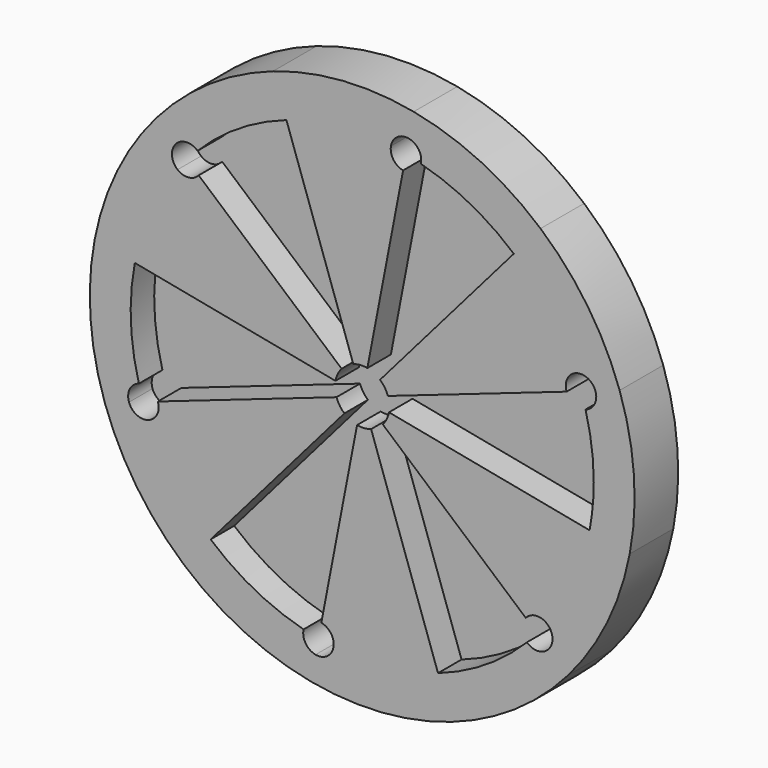
from build123d import *

# Parameters (mm, degrees)
F1_DEPTH = 12.7
F2_R     = 63.5
F3_DEPTH = 5.842


# Not quite as in the source:
# - a feature names something its author has since deleted; it is built from what else it names


with BuildPart() as f1:
    # F0 (on Front) → F1 (new body)
    with BuildSketch(Plane.XZ):
        with BuildLine():
            Line((54.3616852417, 18.8314401648), (60.0018600902, 20.785254045))
            ThreePointArc((60.0018600902, 20.785254045), (52.5777266824, 35.6066378209), (41.57050809, 48.0014880722))
            Line((41.57050809, 48.0014880722), (35.3349318765, 40.8012648613))
            ThreePointArc((35.3349318765, 40.8012648613), (43.6698276291, 31.7213930943), (49.7275527638, 20.9874038681))
            ThreePointArc((49.7275527638, 20.9874038681), (52.5015720726, 20.8916190072), (54.3616852417, 18.8314401648))
        make_face()
        with BuildLine():
            Line((35.3349318765, 40.8012648613), (41.57050809, 48.0014880722))
            ThreePointArc((41.57050809, 48.0014880722), (27.7303280697, 57.1251162375), (12.000372018, 62.3557621349))
            Line((12.000372018, 62.3557621349), (10.8723370483, 56.4943204943))
            ThreePointArc((10.8723370483, 56.4943204943), (12.9421077904, 55.2668436539), (13.7563162153, 53.0023978147))
            ThreePointArc((13.7563162153, 53.0023978147), (13.7342201731, 52.6065963274), (13.6682066443, 52.2157136514))
            ThreePointArc((13.6682066443, 52.2157136514), (25.1574900679, 47.7535477057), (35.3349318765, 40.8012648613))
        make_face()
        with BuildLine():
            Line((10.8723370483, 56.4943204943), (12.000372018, 62.3557621349))
            ThreePointArc((12.000372018, 62.3557621349), (-4.5473895551, 63.3369658907), (-20.785254045, 60.0018600902))
            Line((-20.785254045, 60.0018600902), (-17.6674659382, 51.0015810767))
            ThreePointArc((-17.6674659382, 51.0015810767), (-5.6366184485, 53.6798766529), (6.6881514727, 53.5590258955))
            ThreePointArc((6.6881514727, 53.5590258955), (8.1581132499, 55.9135046571), (10.8723370483, 56.4943204943))
        make_face()
        with BuildLine():
            Line((-17.6674659382, 51.0015810767), (-20.785254045, 60.0018600902))
            ThreePointArc((-20.785254045, 60.0018600902), (-35.6066378209, 52.5777266824), (-48.0014880722, 41.57050809))
            Line((-48.0014880722, 41.57050809), (-43.4893481934, 37.6628803295))
            ThreePointArc((-43.4893481934, 37.6628803295), (-40.9974571589, 38.8855155725), (-38.3860311767, 37.9448710039))
            ThreePointArc((-38.3860311767, 37.9448710039), (-28.7770404, 45.6637993471), (-17.6674659382, 51.0015810767))
        make_face()
        with BuildLine():
            Line((-43.4893481934, 37.6628803295), (-48.0014880722, 41.57050809))
            ThreePointArc((-48.0014880722, 41.57050809), (-57.1251162375, 27.7303280697), (-62.3557621349, 12.000372018))
            Line((-62.3557621349, 12.000372018), (-53.0023978147, 10.2003162153))
            ThreePointArc((-53.0023978147, 10.2003162153), (-49.3064460776, 21.9584835586), (-43.0394012911, 32.5716220275))
            ThreePointArc((-43.0394012911, 32.5716220275), (-44.3434588227, 35.0218856499), (-43.4893481934, 37.6628803295))
        make_face()
        with BuildLine():
            Line((-53.0023978147, 10.2003162153), (-62.3557621349, 12.000372018))
            ThreePointArc((-62.3557621349, 12.000372018), (-63.3369658907, -4.5473895551), (-60.0018600902, -20.785254045))
            Line((-60.0018600902, -20.785254045), (-54.3616852417, -18.8314401648))
            ThreePointArc((-54.3616852417, -18.8314401648), (-54.1745729045, -16.062081604), (-52.054237821, -14.2708426476))
            ThreePointArc((-52.054237821, -14.2708426476), (-53.9345304679, -2.0897483586), (-53.0023978147, 10.2003162153))
        make_face()
        with BuildLine():
            ThreePointArc((-60.0018600902, -20.785254045), (-52.5777266824, -35.6066378209), (-41.57050809, -48.0014880722))
            Line((-41.57050809, -48.0014880722), (-35.3349318765, -40.8012648613))
            ThreePointArc((-35.3349318765, -40.8012648613), (-43.6698276292, -31.7213930943), (-49.7275527638, -20.9874038681))
            ThreePointArc((-49.7275527638, -20.9874038681), (-52.5015720726, -20.8916190072), (-54.3616852417, -18.8314401648))
            Line((-54.3616852417, -18.8314401648), (-60.0018600902, -20.785254045))
        make_face()
        with BuildLine():
            ThreePointArc((-41.57050809, -48.0014880722), (-27.7303280697, -57.1251162375), (-12.000372018, -62.3557621349))
            Line((-12.000372018, -62.3557621349), (-10.8723370483, -56.4943204943))
            ThreePointArc((-10.8723370483, -56.4943204943), (-13.1771157456, -54.9475971764), (-13.6682066443, -52.2157136514))
            ThreePointArc((-13.6682066443, -52.2157136514), (-25.1574900679, -47.7535477057), (-35.3349318765, -40.8012648613))
            Line((-35.3349318765, -40.8012648613), (-41.57050809, -48.0014880722))
        make_face()
        with BuildLine():
            ThreePointArc((-12.000372018, -62.3557621349), (4.5473895551, -63.3369658907), (20.785254045, -60.0018600902))
            Line((20.785254045, -60.0018600902), (17.6674659382, -51.0015810767))
            ThreePointArc((17.6674659382, -51.0015810767), (5.6366184485, -53.6798766529), (-6.6881514727, -53.5590258955))
            ThreePointArc((-6.6881514727, -53.5590258955), (-8.1581132499, -55.9135046571), (-10.8723370483, -56.4943204943))
            Line((-10.8723370483, -56.4943204943), (-12.000372018, -62.3557621349))
        make_face()
        with BuildLine():
            ThreePointArc((20.785254045, -60.0018600902), (35.6066378209, -52.5777266824), (48.0014880722, -41.57050809))
            Line((48.0014880722, -41.57050809), (43.4893481934, -37.6628803295))
            ThreePointArc((43.4893481934, -37.6628803295), (40.9974571589, -38.8855155725), (38.3860311767, -37.9448710039))
            ThreePointArc((38.3860311767, -37.9448710039), (28.7770404, -45.6637993471), (17.6674659382, -51.0015810767))
            Line((17.6674659382, -51.0015810767), (20.785254045, -60.0018600902))
        make_face()
        with BuildLine():
            ThreePointArc((48.0014880722, -41.57050809), (57.1251162375, -27.7303280697), (62.3557621349, -12.000372018))
            Line((62.3557621349, -12.000372018), (53.0023978147, -10.2003162153))
            ThreePointArc((53.0023978147, -10.2003162153), (49.3064460776, -21.9584835586), (43.0394012911, -32.5716220275))
            ThreePointArc((43.0394012911, -32.5716220275), (44.0109337807, -33.8041930262), (44.3572648613, -35.3349318765))
            ThreePointArc((44.3572648613, -35.3349318765), (44.1332282712, -36.5771701127), (43.4893481934, -37.6628803295))
            Line((43.4893481934, -37.6628803295), (48.0014880722, -41.57050809))
        make_face()
        with BuildLine():
            ThreePointArc((62.3557621349, -12.000372018), (63.2132932838, -6.0274001208), (63.5, 0))
            ThreePointArc((63.5, 0), (62.6193584913, 10.5387827635), (60.0018600902, 20.785254045))
            Line((60.0018600902, 20.785254045), (54.3616852417, 18.8314401648))
            ThreePointArc((54.3616852417, 18.8314401648), (54.5082651522, 18.257637773), (54.5575810767, 17.6674659382))
            ThreePointArc((54.5575810767, 17.6674659382), (53.864130935, 15.5577398165), (52.054237821, 14.2708426476))
            ThreePointArc((52.054237821, 14.2708426476), (53.4926542218, 7.1997617534), (53.975, 0))
            ThreePointArc((53.975, 0), (53.7312992912, -5.1232901027), (53.0023978147, -10.2003162153))
            Line((53.0023978147, -10.2003162153), (62.3557621349, -12.000372018))
        make_face()
        with BuildLine():
            ThreePointArc((-6.2355762135, 1.2000372018), (-5.7125116237, 2.773032807), (-4.8001488072, 4.157050809))
            Line((-4.8001488072, 4.157050809), (-38.1131815293, 33.0069834234))
            ThreePointArc((-38.1131815293, 33.0069834234), (-40.4882186348, 31.7927379151), (-43.0394012911, 32.5716220275))
            ThreePointArc((-43.0394012911, 32.5716220275), (-49.3064460776, 21.9584835586), (-53.0023978147, 10.2003162153))
            Line((-53.0023978147, 10.2003162153), (-6.2355762135, 1.2000372018))
        make_face()
        with BuildLine():
            ThreePointArc((-6.6881514727, -53.5590258955), (5.6366184485, -53.6798766529), (17.6674659382, -51.0015810767))
            Line((17.6674659382, -51.0015810767), (2.0785254045, -6.000186009))
            ThreePointArc((2.0785254045, -6.000186009), (0.4547389555, -6.3336965891), (-1.2000372018, -6.2355762135))
            Line((-1.2000372018, -6.2355762135), (-9.5282953823, -49.5104751351))
            ThreePointArc((-9.5282953823, -49.5104751351), (-7.4585246403, -50.7379519754), (-6.6443162153, -53.0023978147))
            ThreePointArc((-6.6443162153, -53.0023978147), (-6.6552919682, -53.2815735435), (-6.6881514727, -53.5590258955))
        make_face()
        with BuildLine():
            Line((-35.3349318765, -40.8012648613), (-4.157050809, -4.8001488072))
            ThreePointArc((-4.157050809, -4.8001488072), (-5.2577726682, -3.5606637821), (-6.000186009, -2.0785254045))
            Line((-6.000186009, -2.0785254045), (-47.6414769116, -16.5034917117))
            ThreePointArc((-47.6414769116, -16.5034917117), (-47.4948970012, -17.0772941035), (-47.4455810767, -17.6674659382))
            ThreePointArc((-47.4455810767, -17.6674659382), (-48.0710878861, -19.681751335), (-49.7275527638, -20.9874038681))
            ThreePointArc((-49.7275527638, -20.9874038681), (-43.6698276292, -31.7213930943), (-35.3349318765, -40.8012648613))
        make_face()
        with BuildLine():
            ThreePointArc((6.6881514727, 53.5590258955), (-5.6366184485, 53.6798766529), (-17.6674659382, 51.0015810767))
            Line((-17.6674659382, 51.0015810767), (-2.0785254045, 6.000186009))
            ThreePointArc((-2.0785254045, 6.000186009), (-0.4547389555, 6.3336965891), (1.2000372018, 6.2355762135))
            Line((1.2000372018, 6.2355762135), (9.5282953823, 49.5104751351))
            ThreePointArc((9.5282953823, 49.5104751351), (7.2892093729, 50.9601948492), (6.6881514727, 53.5590258955))
        make_face()
        with BuildLine():
            ThreePointArc((43.0394012911, -32.5716220275), (49.3064460776, -21.9584835586), (53.0023978147, -10.2003162153))
            Line((53.0023978147, -10.2003162153), (6.2355762135, -1.2000372018))
            ThreePointArc((6.2355762135, -1.2000372018), (5.7125116237, -2.773032807), (4.8001488072, -4.157050809))
            Line((4.8001488072, -4.157050809), (38.1131815293, -33.0069834234))
            ThreePointArc((38.1131815293, -33.0069834234), (40.4882186348, -31.7927379151), (43.0394012911, -32.5716220275))
        make_face()
        with BuildLine():
            ThreePointArc((49.7275527638, 20.9874038681), (43.6698276291, 31.7213930943), (35.3349318765, 40.8012648613))
            Line((35.3349318765, 40.8012648613), (4.157050809, 4.8001488072))
            ThreePointArc((4.157050809, 4.8001488072), (5.2577726682, 3.5606637821), (6.000186009, 2.0785254045))
            Line((6.000186009, 2.0785254045), (47.6414769116, 16.5034917117))
            ThreePointArc((47.6414769116, 16.5034917117), (47.7774280077, 19.1674569341), (49.7275527638, 20.9874038681))
        make_face()
    extrude(amount=F1_DEPTH)

    # F2 (on Front) → F3 (join)
    with BuildSketch(Plane.XZ):
        Circle(F2_R)
    extrude(amount=F3_DEPTH)


solid = f1.part
